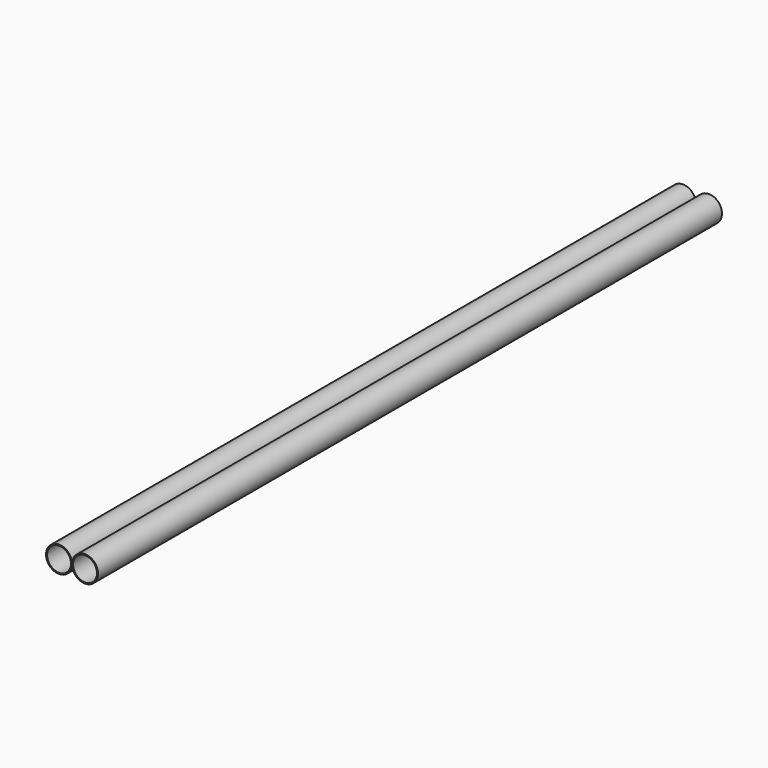
from build123d import *

# Parameters (mm, degrees)
F0_R     = 2.5
F1_DEPTH = 150
F2_T     = -0.2
F2_2_T   = -0.2


with BuildPart() as f1:
    # F0 (on Front) → F1 (new body)
    with BuildSketch(Plane.XZ):
        with Locations((-2.5, 0)):
            Circle(F0_R)
    extrude(amount=F1_DEPTH)

    # F2
    f2_openings = [f1.faces().sort_by_distance(p)[0] for p in [
        (-2.5, -150, 0),
    ]]
    offset(amount=F2_T, openings=f2_openings)


with BuildPart() as f1b:
    # F0 (on Front) → F1, piece 2 (new body)
    with BuildSketch(Plane.XZ):
        with BuildLine():
            ThreePointArc((5, 0), (2.5, 2.5), (0, 0))
            ThreePointArc((0, 0), (2.5, -2.5), (5, 0))
        make_face()
    extrude(amount=F1_DEPTH)

    # F2#2
    f2_2_openings = [f1b.faces().sort_by_distance(p)[0] for p in [
        (2.5, -150, 0),
    ]]
    offset(amount=F2_2_T, openings=f2_2_openings)


solid = Compound([f1.part, f1b.part])
